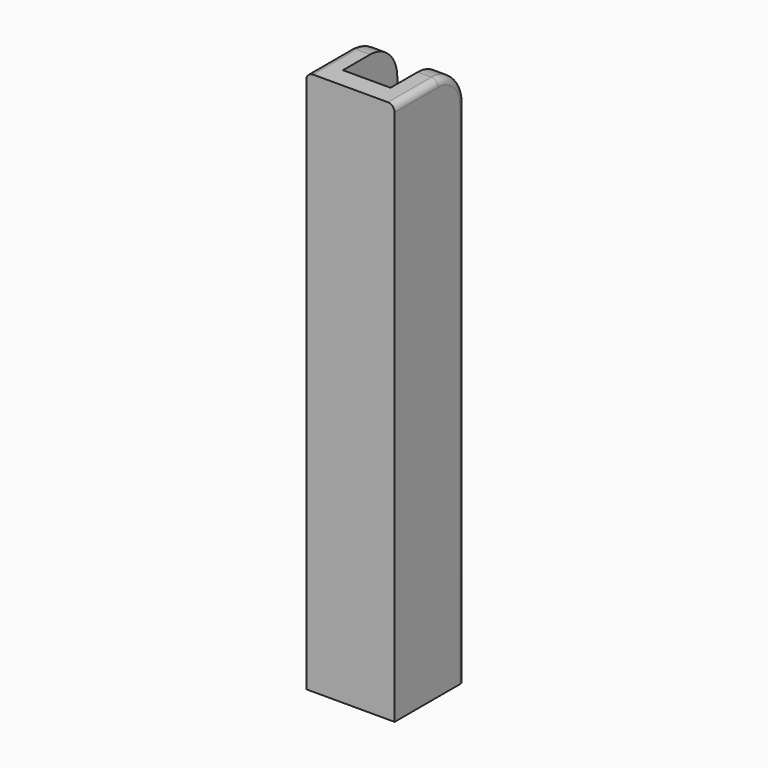
from build123d import *

# Parameters (mm, degrees)
F1_DEPTH = 13
F2_R     = 5
F3_R     = 1
F4_W     = 7
F4_H     = 80.0645950389
F5_DEPTH = 10


with BuildPart() as f1:
    # F0 (on Right) → F1 (new body)
    with BuildSketch(Plane.YZ):
        Polygon((-56.8815148667, 19.1431619976), (-69.8815148667, 19.1431619976), (-69.8815148667, -60.8568380024), (-56.8815148667, -60.8568380024), (-56.8815148667, -47.8568380024), align=None)
    extrude(amount=F1_DEPTH)

    # F2
    f2_edges = [f1.edges().sort_by_distance(p)[0] for p in [
        (6.5, -56.881515, 19.143162),
    ]]
    fillet(f2_edges, radius=F2_R)

    # F3
    f3_edges = [f1.edges().sort_by_distance(p)[0] for p in [
        (0, -56.881515, -23.356838),
        (13, -56.881515, -23.356838),
        (0, -65.881515, 19.143162),
        (13, -65.881515, 19.143162),
        (0, -58.345981, 17.678696),
        (13, -58.345981, 17.678696),
    ]]
    fillet(f3_edges, radius=F3_R)

    # F4 (on face) → F5 (cut)
    with BuildSketch(Plane(origin=(0, -56.8815148667, 0), x_dir=(-1, 0, 0), z_dir=(0, 1, 0))):
        with Locations((-6.5, -20.824540483)):
            Rectangle(F4_W, F4_H)
    extrude(amount=-F5_DEPTH, mode=Mode.SUBTRACT)


solid = f1.part
